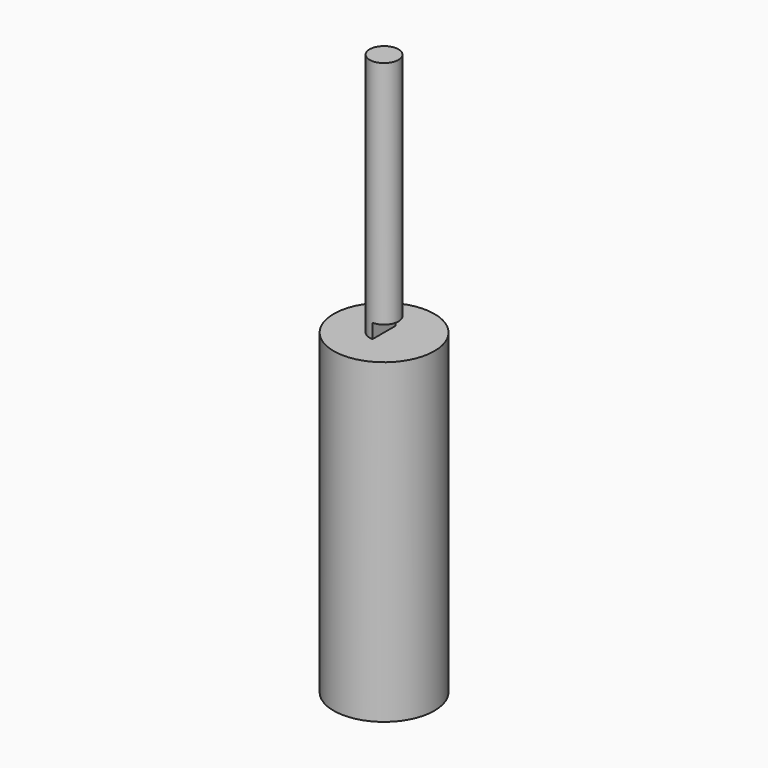
from build123d import *

# Parameters (mm, degrees)
F0_R     = 3.5
F1_DEPTH = 22
F2_START = 1
F2_DEPTH = 16
F3_DEPTH = 1


# Not quite as in the source:
# - a feature names something its author has since deleted; it is built from what else it names


with BuildPart() as f1:
    # F0 (on Top) → F1 (new body)
    with BuildSketch(Plane.XY):
        Circle(F0_R)
        with BuildLine():
            ThreePointArc((0, 1), (0.7071067812, 0.7071067812), (1, 0))
            ThreePointArc((1, 0), (0.7071067812, -0.7071067812), (0, -1))
            ThreePointArc((0, -1), (-1, 0), (0, 1))
        make_face(mode=Mode.SUBTRACT)
        with BuildLine():
            Line((0, 0), (0, 1))
            ThreePointArc((0, 1), (-1, 0), (0, -1))
            Line((0, -1), (0, 0))
        make_face()
        with BuildLine():
            ThreePointArc((0, -1), (0.7071067812, -0.7071067812), (1, 0))
            ThreePointArc((1, 0), (0.7071067812, 0.7071067812), (0, 1))
            Line((0, 1), (0, 0))
            Line((0, 0), (0, -1))
        make_face()
    extrude(amount=-F1_DEPTH)



with BuildPart() as f2:
    # F0 (on Top) → F2 (new body)
    with BuildSketch(Plane.XY.offset(F2_START)):
        with BuildLine():
            Line((0, 0), (0, 1))
            ThreePointArc((0, 1), (-1, 0), (0, -1))
            Line((0, -1), (0, 0))
        make_face()
        with BuildLine():
            ThreePointArc((0, -1), (0.7071067812, -0.7071067812), (1, 0))
            ThreePointArc((1, 0), (0.7071067812, 0.7071067812), (0, 1))
            Line((0, 1), (0, 0))
            Line((0, 0), (0, -1))
        make_face()
    extrude(amount=F2_DEPTH)


with BuildPart() as f1_1:
    add(f1.part)

    add(f2.part)  # F3 merges F2
    # F0 (on Top) → F3 (join)
    with BuildSketch(Plane.XY):
        with BuildLine():
            Line((0, 0), (0, 1))
            ThreePointArc((0, 1), (-1, 0), (0, -1))
            Line((0, -1), (0, 0))
        make_face()
    extrude(amount=F3_DEPTH)


solid = f1_1.part
